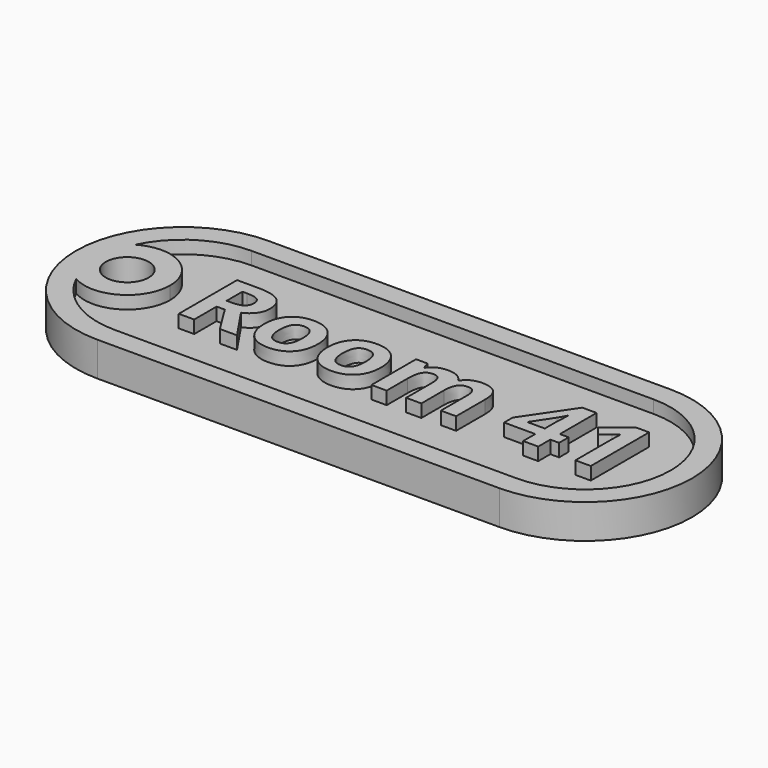
from build123d import *

# Parameters (mm, degrees)
F1_DEPTH     = 4
F3_DEPTH     = 1.5
F5_DEPTH     = 1.5
F6_R         = 2.5
F7_DEPTH     = 25
F8_TEXT_SIZE = 11.935844834
F9_DEPTH     = 1.5


# Not quite as in the source:
# - Text() gives the source's letters only with a copy of the font that has no kerning and outlines rounded to 1/6400 em; it was checked with that copy


with BuildPart() as f1:
    # F0 (on Top) → F1 (new body)
    with BuildSketch(Plane.XY):
        with BuildLine():
            ThreePointArc((12.5, 25), (0, 12.5), (12.5, 0))
            Line((12.5, 0), (59.5057010651, 0))
            ThreePointArc((59.5057010651, 0), (72.0057010651, 12.5), (59.5057010651, 25))
            Line((59.5057010651, 25), (12.5, 25))
        make_face()
    extrude(amount=F1_DEPTH)

    # F2 (on face) → F3 (cut)
    with BuildSketch(Plane.XY.offset(4)):
        with BuildLine():
            Line((59.5057010651, 22.5), (12.5, 22.5))
            ThreePointArc((12.5, 22.5), (2.5, 12.5), (12.5, 2.5))
            Line((12.5, 2.5), (59.5057010651, 2.5))
            ThreePointArc((59.5057010651, 2.5), (69.5057010651, 12.5), (59.5057010651, 22.5))
        make_face()
    extrude(amount=-F3_DEPTH, mode=Mode.SUBTRACT)

    # F4 (on face) → F5 (join)
    with BuildSketch(Plane.XY.offset(2.5)):
        with BuildLine():
            ThreePointArc((3.4807692308, 8.1810329555), (8.4903660528, 8.1643250902), (11, 12.5))
            ThreePointArc((11, 12.5), (8.4903660528, 16.8356749098), (3.4807692308, 16.8189670445))
            ThreePointArc((3.4807692308, 16.8189670445), (2.5, 12.5), (3.4807692308, 8.1810329555))
        make_face()
    extrude(amount=F5_DEPTH)

    # F6 (on face) → F7 (cut)
    with BuildSketch(Plane.XY.offset(4)):
        with Locations((6, 12.5)):
            Circle(F6_R)
    extrude(amount=-F7_DEPTH, mode=Mode.SUBTRACT)

    # F8 (on face) → F9 (join)
    with BuildSketch(Plane.XY.offset(2.5)):
        with Locations((14.0350442667, 8.6346905943)):
            Text('Room 41', F8_TEXT_SIZE, font='Open Sans', font_style=FontStyle.BOLD, text_align=(TextAlign.LEFT, TextAlign.BOTTOM))
    extrude(amount=F9_DEPTH)


solid = f1.part
